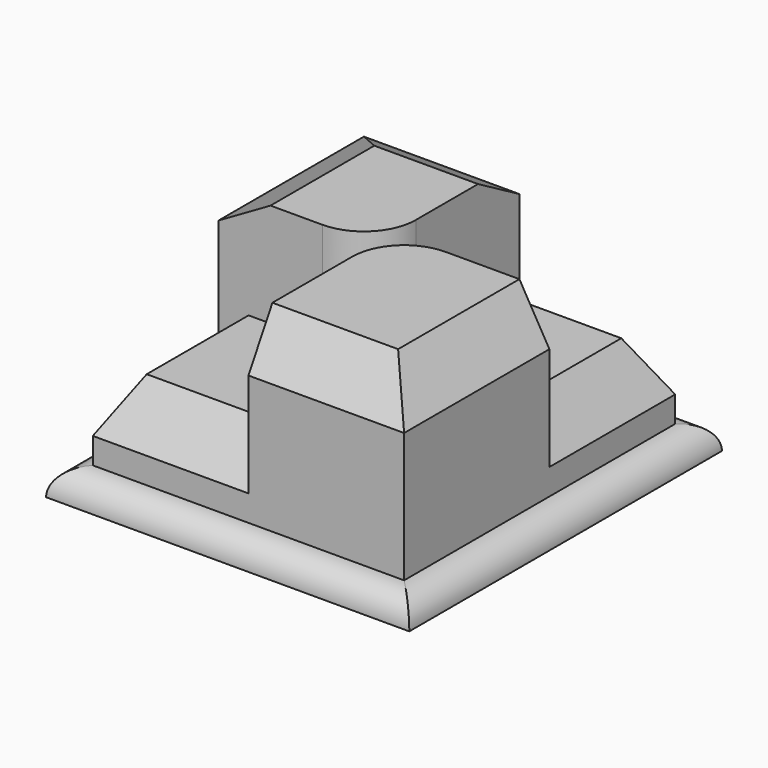
from build123d import *

# Parameters (mm, degrees)
F0_W        = 88.8999994576
F0_H        = 95.6510528922
F1_DEPTH    = 6.35
F2_DEPTH    = 25.4
F3_DEPTH    = 50.8
F4_R        = 6.34999
F5_SIZE2    = 7.3323484187
F5_SIZE     = 12.7
F6_C1_SIZE2 = 12.7
F6_C1_SIZE  = 7.3323484187
F6_C2_SIZE2 = 7.3323484187
F6_C2_SIZE  = 12.7
F6_C3_SIZE2 = 12.7
F6_C3_SIZE  = 7.3323484187
F6_C4_SIZE2 = 7.3323484187
F6_C4_SIZE  = 12.7


# Not quite as in the source:
# - a fillet or chamfer is up to 0.001 mm smaller than in the source, because OpenCascade refuses the exact size


with BuildPart() as f1:
    # F0 (on Top) → F1 (new body)
    with BuildSketch(Plane.XY):
        Rectangle(F0_W, F0_H)
        Polygon((-2.712e-07, 41.4755269885), (38.0999997288, 41.4755269885), (38.0999997288, 2.9744735539), (38.0999997288, -41.4755264461), (-2.712e-07, -41.4755264461), (-38.1000002712, -41.4755264461), (-38.1000002712, -2.9744730115), (-38.1000002712, 41.4755269885), align=None, mode=Mode.SUBTRACT)
    extrude(amount=F1_DEPTH)

    # F0 (on Top) → F2 (join)
    with BuildSketch(Plane.XY):
        with BuildLine():
            Line((38.0999997288, 2.9744735539), (38.0999997288, 41.4755269885))
            Line((38.0999997288, 41.4755269885), (-2.712e-07, 41.4755269885))
            Line((-2.712e-07, 41.4755269885), (-2.712e-07, 9.7255269885))
            ThreePointArc((-2.712e-07, 9.7255269885), (-3.7197441501, 0.7452708674), (-12.7000002712, -2.9744730115))
            Line((-12.7000002712, -2.9744730115), (-38.1000002712, -2.9744730115))
            Line((-38.1000002712, -2.9744730115), (-38.1000002712, -41.4755264461))
            Line((-38.1000002712, -41.4755264461), (-2.712e-07, -41.4755264461))
            Line((-2.712e-07, -41.4755264461), (-2.712e-07, -9.7255264461))
            ThreePointArc((-2.712e-07, -9.7255264461), (3.7197436077, -0.745270325), (12.6999997288, 2.9744735539))
            Line((12.6999997288, 2.9744735539), (38.0999997288, 2.9744735539))
        make_face()
    extrude(amount=F2_DEPTH)

    # F0 (on Top) → F3 (join)
    with BuildSketch(Plane.XY):
        with BuildLine():
            Line((-2.712e-07, 9.7255269885), (-2.712e-07, 41.4755269885))
            Line((-2.712e-07, 41.4755269885), (-38.1000002712, 41.4755269885))
            Line((-38.1000002712, 41.4755269885), (-38.1000002712, -2.9744730115))
            Line((-38.1000002712, -2.9744730115), (-12.7000002712, -2.9744730115))
            ThreePointArc((-12.7000002712, -2.9744730115), (-3.7197441501, 0.7452708674), (-2.712e-07, 9.7255269885))
        make_face()
        with BuildLine():
            Line((38.0999997288, -41.4755264461), (38.0999997288, 2.9744735539))
            Line((38.0999997288, 2.9744735539), (12.6999997288, 2.9744735539))
            ThreePointArc((12.6999997288, 2.9744735539), (3.7197436077, -0.745270325), (-2.712e-07, -9.7255264461))
            Line((-2.712e-07, -9.7255264461), (-2.712e-07, -41.4755264461))
            Line((-2.712e-07, -41.4755264461), (38.0999997288, -41.4755264461))
        make_face()
    extrude(amount=F3_DEPTH)

    # F4 (radius 6.35 in the source; OpenCascade refuses exactly that, so slightly less here)
    f4_edges = [f1.edges().sort_by_distance(p)[0] for p in [
        (44.45, 0, 6.35),
        (0, -47.825526, 6.35),
        (0, 47.825526, 6.35),
        (-44.45, 0, 6.35),
    ]]
    fillet(f4_edges, radius=F4_R)

    # F5
    f5_edges = [f1.edges().sort_by_distance(p)[0] for p in [
        (38.1, 22.225, 25.4),
        (19.05, 41.475527, 25.4),
        (-38.1, -22.225, 25.4),
        (-19.05, -41.475526, 25.4),
    ]]
    chamfer(f5_edges, length=F5_SIZE, length2=F5_SIZE2)

    # F6: chamfer of 12.7 x 7.3323484187 on 4 edges, made by hand

    # F6_c1
    f6_c1_edges = [f1.edges().sort_by_distance(p)[0] for p in [
        (-19.0500002712, 41.4755269885, 50.8),
    ]]
    f6_c1_side = f1.faces().sort_by_distance((-19.0500002712, 41.4755269885, 50.6533530316))[0]
    chamfer(f6_c1_edges, length=F6_C1_SIZE, length2=F6_C1_SIZE2, reference=f6_c1_side)

    # F6_c2
    f6_c2_edges = [f1.edges().sort_by_distance(p)[0] for p in [
        (38.0999997288, -19.2505264461, 50.8),
    ]]
    f6_c2_side = f1.faces().sort_by_distance((38.0999997288, -19.2505264461, 50.6533530316))[0]
    chamfer(f6_c2_edges, length=F6_C2_SIZE, length2=F6_C2_SIZE2, reference=f6_c2_side)

    # F6_c3
    f6_c3_edges = [f1.edges().sort_by_distance(p)[0] for p in [
        (-38.1000002712, 12.9005269885, 50.8),
    ]]
    f6_c3_side = f1.faces().sort_by_distance((-38.1000002712, 12.9005269885, 50.6533530316))[0]
    chamfer(f6_c3_edges, length=F6_C3_SIZE, length2=F6_C3_SIZE2, reference=f6_c3_side)

    # F6_c4
    f6_c4_edges = [f1.edges().sort_by_distance(p)[0] for p in [
        (15.3838255194, -41.4755264461, 50.8),
    ]]
    f6_c4_side = f1.faces().sort_by_distance((15.3838255194, -41.4755264461, 50.6533530316))[0]
    chamfer(f6_c4_edges, length=F6_C4_SIZE, length2=F6_C4_SIZE2, reference=f6_c4_side)


solid = f1.part
